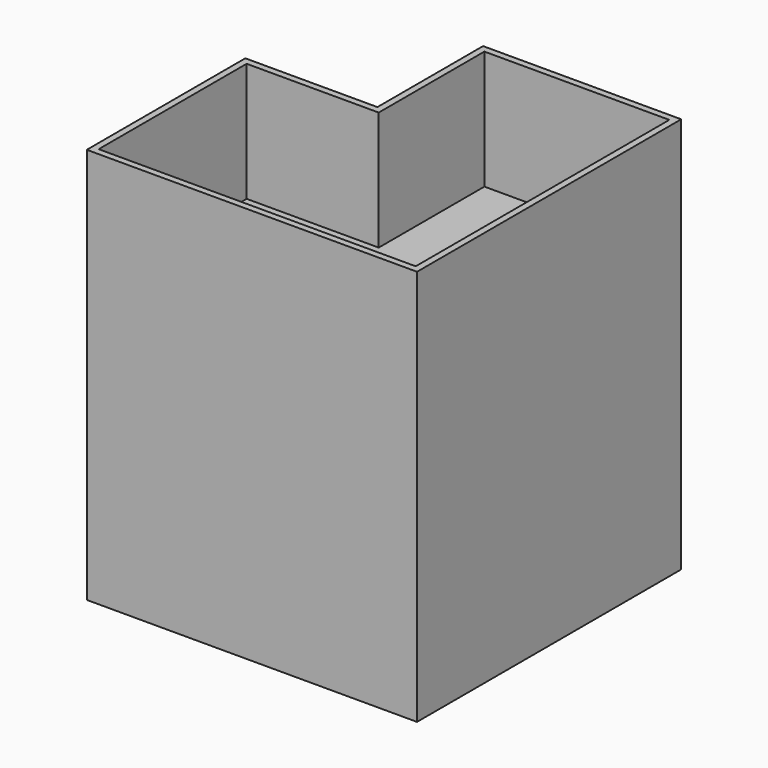
from build123d import *

# Parameters (mm, degrees)
F1_DEPTH = 600
F2_T     = -10
F5_DEPTH = 10


# Not quite as in the source:
# - a feature names something its author has since deleted; it is built from what else it names


with BuildPart() as f1:
    # F0 (on Top) → F1 (new body)
    with BuildSketch(Plane.XY):
        Polygon((-250, -250), (250, -250), (250, 250), (-50, 250), (-50, 50), (-250, 50), align=None)
    extrude(amount=F1_DEPTH)

    # F2
    f2_openings = [f1.faces().sort_by_distance(p)[0] for p in [
        (28.571429, -28.571429, 600),
    ]]
    offset(amount=F2_T, openings=f2_openings, kind=Kind.INTERSECTION)

    # F4 (on offset) → F5 (join)
    with BuildSketch(Plane.XY.offset(410)):
        Polygon((-240, 40), (-240, -240), (240, -240), (240, 240), (-40, 240), (-40, 40), align=None)
    extrude(amount=F5_DEPTH)


solid = f1.part
